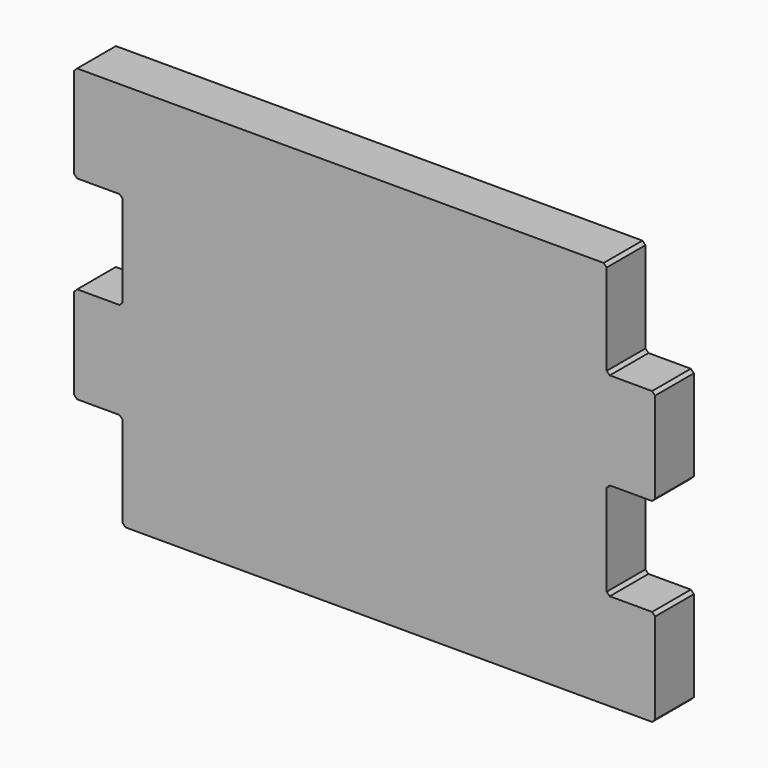
from build123d import *

# Parameters (mm, degrees)
F1_DEPTH = 12.7
F2_SIZE  = 0.79375


# Not quite as in the source:
# - a feature names something its author has since deleted; it is built from what else it names


with BuildPart() as f1:
    # F0 (on Front) → F1 (new body)
    with BuildSketch(Plane.XZ):
        Polygon((-63.5, 25.4508), (-63.5, 0), (76.2, 0), (76.2, 25.4), (63.5, 25.4), (63.5, 51.0032), (76.2, 51.0032), (76.2, 76.4032), (63.5, 76.4032), (63.5, 101.854), (-76.2, 101.854), (-76.2, 76.454), (-63.5, 76.454), (-63.5, 50.8508), (-76.2, 50.8508), (-76.2, 25.4508), align=None)
    extrude(amount=F1_DEPTH)

    # F2
    f2_edges = [f1.edges().sort_by_distance(p)[0] for p in [
        (-63.5, -6.35, 76.454),
        (-63.5, -6.35, 50.8508),
        (-63.5, -6.35, 25.4508),
        (-63.5, -6.35, 0),
        (63.5, -6.35, 101.854),
        (76.2, -6.35, 76.4032),
        (63.5, -6.35, 76.4032),
        (63.5, -6.35, 25.4),
        (76.2, -6.35, 25.4),
        (76.2, -6.35, 51.0032),
        (63.5, -6.35, 51.0032),
        (-76.2, -6.35, 50.8508),
        (-76.2, -6.35, 25.4508),
        (76.2, -6.35, 0),
        (-76.2, -6.35, 101.854),
        (-76.2, -6.35, 76.454),
    ]]
    chamfer(f2_edges, length=F2_SIZE)


solid = f1.part
